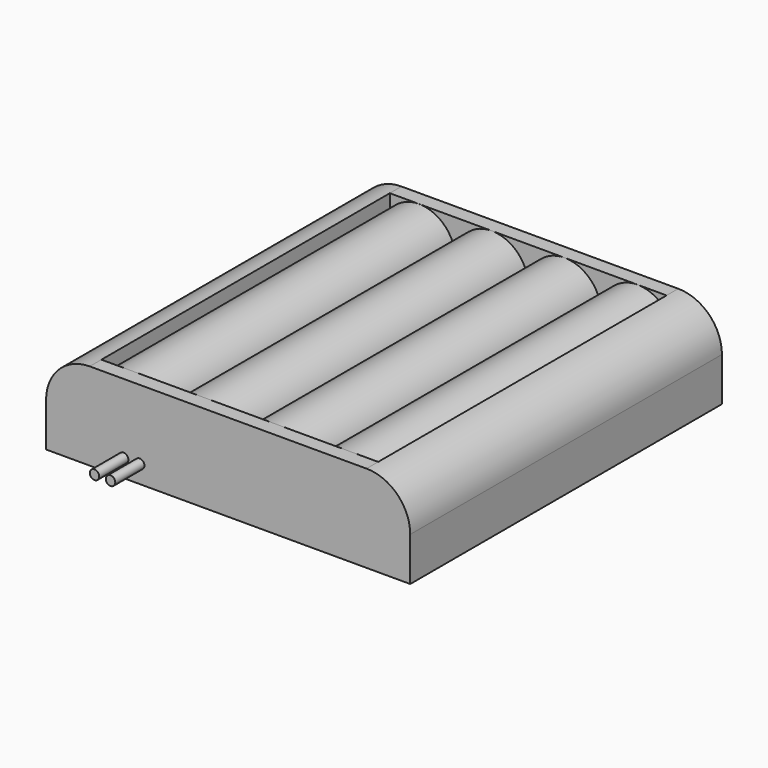
from build123d import *

# Parameters (mm, degrees)
F0_W     = 50
F0_H     = 53.5
F1_DEPTH = 12
F2_R     = 6
F3_T     = -2
F4_R     = 1.5
F5_DEPTH = 3
F6_R     = 0.65
F7_DEPTH = 5
F8_R     = 5
F9_DEPTH = 49.5


# Not quite as in the source:
# - a shell that OpenCascade refuses in one call is made with other operations: the cavity is built on its own and cut out


with BuildPart() as f1:
    # F0 (on Top) → F1 (new body)
    with BuildSketch(Plane.XY):
        Rectangle(F0_W, F0_H)
    extrude(amount=F1_DEPTH)

    # F2
    f2_edges = [f1.edges().sort_by_distance(p)[0] for p in [
        (25, 0, 12),
        (-25, 0, 12),
    ]]
    fillet(f2_edges, radius=F2_R)

    # F3: a shell. OpenCascade refuses it in one call, so the cavity is built on its own and cut out:
    # the body offset inwards by the wall thickness, plus a prism from it out through each open face.
    f3_core = offset(f1.part, amount=F3_T, mode=Mode.PRIVATE)
    f3_exits = [f3_core.faces().sort_by_distance(p)[0] for p in [
        (0, 0, 10),
    ]]
    add(f3_core, mode=Mode.SUBTRACT)
    extrude(f3_exits, amount=-F3_T, mode=Mode.SUBTRACT)

    # F4 (on face) → F5 (cut)
    with BuildSketch(Plane(origin=(0, 0, 0), x_dir=(1, 0, 0), z_dir=(0, 0, -1))):
        with Locations((-18.5, 0)):
            Circle(F4_R)
        with Locations((18.5, 0)):
            Circle(F4_R)
    extrude(amount=-F5_DEPTH, mode=Mode.SUBTRACT)

    # F6 (on face) → F7 (join)
    with BuildSketch(Plane.XZ.offset(26.75)):
        with Locations((-14.35, 2.45)):
            Circle(F6_R)
        with Locations((-12.15, 2.45)):
            Circle(F6_R)
    extrude(amount=F7_DEPTH)


with BuildPart() as f9:
    # F8 (on face) → F9 (new body, through all)
    with BuildSketch(Plane.XZ.offset(-24.75)):
        with Locations((-15, 7)):
            Circle(F8_R)
    extrude(amount=F9_DEPTH)


with BuildPart() as f9b:
    # F8 (on face) → F9, piece 2 (new body, through all)
    with BuildSketch(Plane.XZ.offset(-24.75)):
        with BuildLine():
            ThreePointArc((20, 7), (15, 12), (10, 7))
            ThreePointArc((10, 7), (15, 2), (20, 7))
        make_face()
    extrude(amount=F9_DEPTH)


with BuildPart() as f9c:
    # F8 (on face) → F9, piece 3 (new body, through all)
    with BuildSketch(Plane.XZ.offset(-24.75)):
        with BuildLine():
            ThreePointArc((10, 7), (5, 12), (0, 7))
            ThreePointArc((0, 7), (5, 2), (10, 7))
        make_face()
    extrude(amount=F9_DEPTH)


with BuildPart() as f9d:
    # F8 (on face) → F9, piece 4 (new body, through all)
    with BuildSketch(Plane.XZ.offset(-24.75)):
        with BuildLine():
            ThreePointArc((0, 7), (-5, 12), (-10, 7))
            ThreePointArc((-10, 7), (-5, 2), (0, 7))
        make_face()
    extrude(amount=F9_DEPTH)


solid = Compound([f1.part, f9.part, f9b.part, f9c.part, f9d.part])
